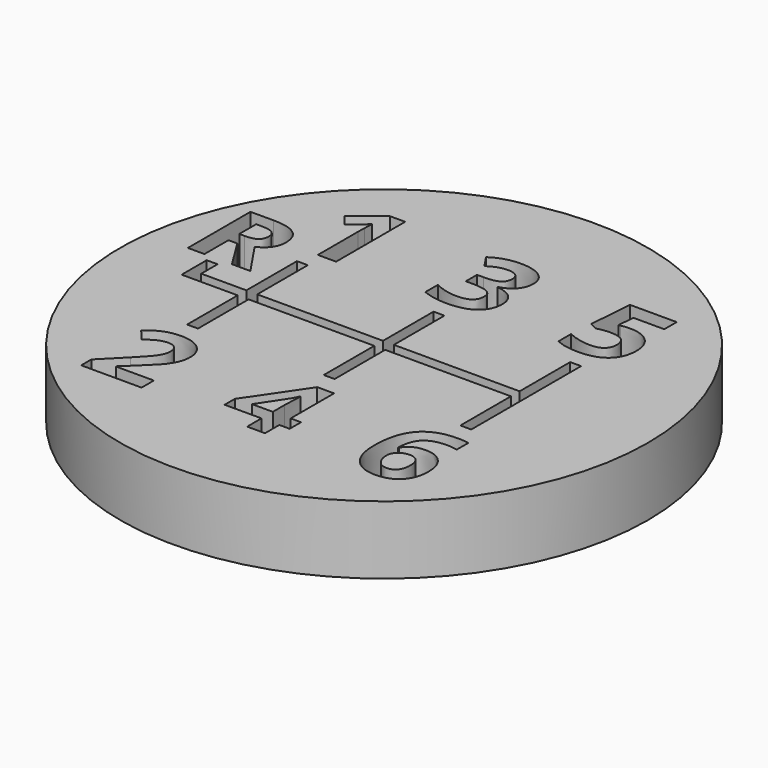
from build123d import *

# Parameters (mm, degrees)
F0_R           = 12.319
F1_DEPTH       = 3.175
F2_TEXT_SIZE   = 5.1152777778
F2_TEXT_SIZE_2 = 5.6444444444
F3_DEPTH       = 1.5875


# Not quite as in the source:
# - a length typed as a fraction of an inch, garbled in the dataset ("3 / 203.2 mm" for 3/8 in), is restored
# - Text() gives the source's letters only with a copy of the font that has no kerning and outlines rounded to 1/6400 em; it was checked with that copy


with BuildPart() as f1:
    # F0 (on Top) → F1 (new body)
    with BuildSketch(Plane.XY):
        Circle(F0_R)
    extrude(amount=F1_DEPTH)

    # F2 (on face) → F3 (cut)
    with BuildSketch(Plane.XY.offset(3.175)):
        Polygon((6.1226557723, 3.20421), (6.1226557723, 0.254), (0.254, 0.254), (0.254, 3.20421), (-0.254, 3.20421), (-0.254, 0.254), (-6.1226557723, 0.254), (-6.1226557723, 3.20421), (-6.6306557723, 3.20421), (-6.6306557723, 0.254), (-8.737471212, 0.254), (-8.737471212, 1.2070476077), (-9.245471212, 1.2070476077), (-9.245471212, -0.254), (-8.991471212, -0.254), (-6.6306557723, -0.254), (-6.6306557723, -3.20421), (-6.1226557723, -3.20421), (-6.1226557723, -0.254), (-0.254, -0.254), (-0.254, -3.20421), (0.254, -3.20421), (0.254, -0.254), (6.1226557723, -0.254), (6.1226557723, -3.20421), (6.6306557723, -3.20421), (6.6306557723, 3.20421), align=None)
        with Locations((-10.8457594065, 1.5353459422)):
            Text('R', F2_TEXT_SIZE, font='Open Sans', font_style=FontStyle.BOLD, text_align=(TextAlign.LEFT, TextAlign.BOTTOM))
        with Locations((-7.82240625, 4.064)):
            Text('1  3  5', F2_TEXT_SIZE_2, font='Open Sans', font_style=FontStyle.BOLD, text_align=(TextAlign.LEFT, TextAlign.BOTTOM))
        with Locations((-7.8594479167, -8.128)):
            Text('2  4  6', F2_TEXT_SIZE_2, font='Open Sans', font_style=FontStyle.BOLD, text_align=(TextAlign.LEFT, TextAlign.BOTTOM))
    extrude(amount=-F3_DEPTH, mode=Mode.SUBTRACT)


solid = f1.part
